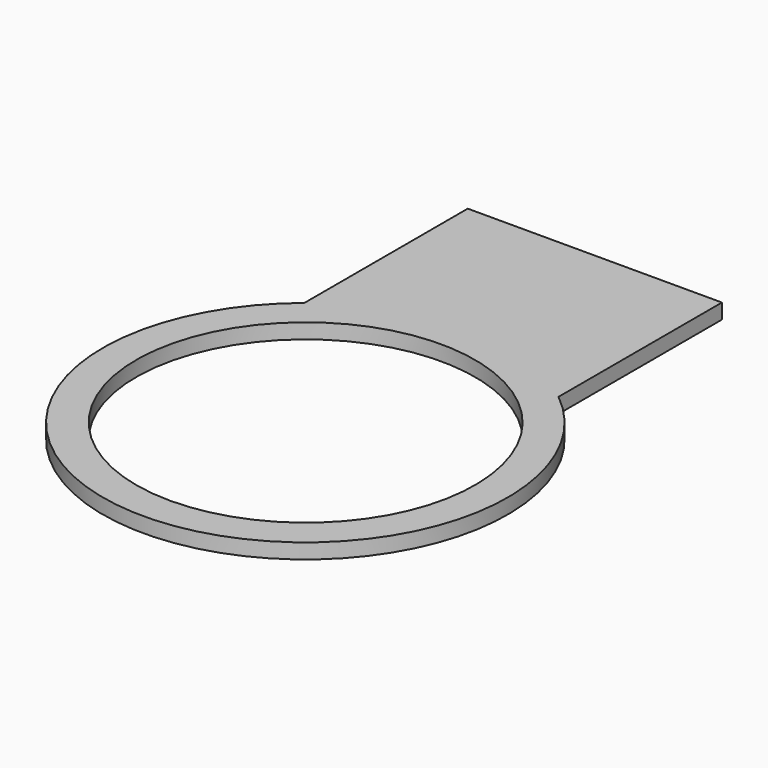
from build123d import *

# Parameters (mm, degrees)
F1_DEPTH = 0.8


# Not quite as in the source:
# - ends of sketch curves that miss each other by under 0.0002 mm in the source are joined


with BuildPart() as f1:
    # F0 (on Top) → F1 (new body, symmetric)
    with BuildSketch(Plane.XY):
        with BuildLine():
            Line((-13.5, 29.939975), (-13.5, 8.264975))
            ThreePointArc((-13.5, 8.264975), (0, -29.989975), (13.500000361, 8.2649754478))
            Line((13.500000361, 8.2649754478), (13.5, 29.939975))
            Line((13.5, 29.939975), (13.5, 29.964975))
            Line((13.5, 29.964975), (13.475, 29.964975))
            Line((13.475, 29.964975), (-13.475, 29.964975))
            Line((-13.475, 29.964975), (-13.5, 29.964975))
            Line((-13.5, 29.964975), (-13.5, 29.939975))
        make_face()
        with BuildLine():
            ThreePointArc((0, 9.564975), (18, -8.435025), (0, -26.435025))
            ThreePointArc((0, -26.435025), (-18, -8.435025), (0, 9.564975))
        make_face(mode=Mode.SUBTRACT)
    extrude(amount=F1_DEPTH, both=True)


solid = f1.part
